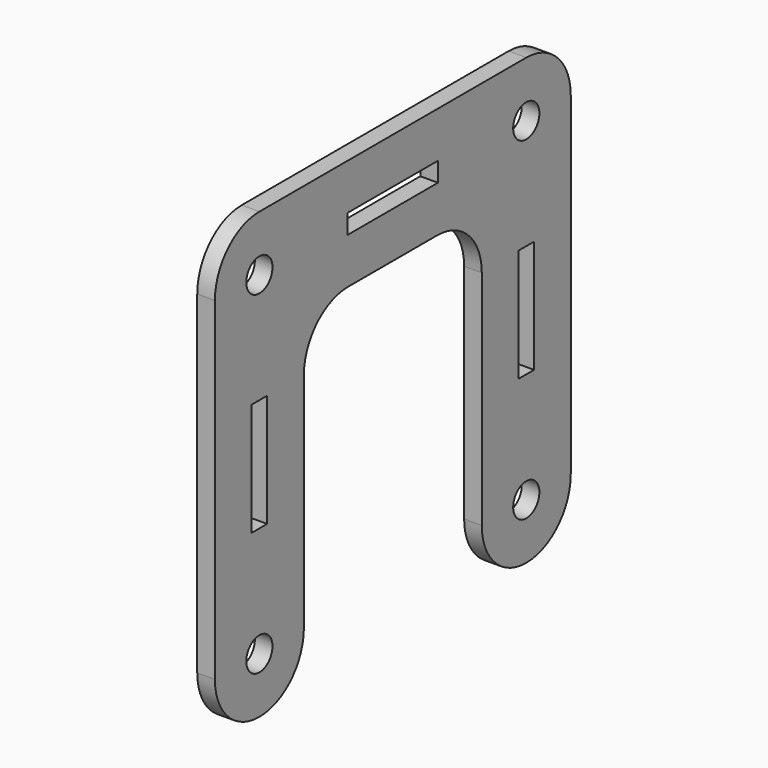
from build123d import *

# Parameters (mm, degrees)
F0_R     = 1.4732
F0_W     = 1.74625
F0_H     = 10.15
F0_W_2   = 10.15
F0_H_2   = 1.74625
F1_DEPTH = 1.5875
F2_R     = 4.99999


# Not quite as in the source:
# - a fillet or chamfer is up to 0.001 mm smaller than in the source, because OpenCascade refuses the exact size
# - a length typed as a fraction of an inch, garbled in the dataset ("3 / 203.2 mm" for 3/8 in), is restored


with BuildPart() as f1:
    # F0 (on Right) → F1 (new body)
    with BuildSketch(Plane.YZ):
        Polygon((20, -20), (20, 20), (-20, 20), (-20, -20), (-10, -20), (-10, 10), (10, 10), (10, -20), align=None)
        with Locations((-15, -15)):
            Circle(F0_R, mode=Mode.SUBTRACT)
        with Locations((15, -15)):
            Circle(F0_R, mode=Mode.SUBTRACT)
        with Locations((-15, 0)):
            Rectangle(F0_W, F0_H, mode=Mode.SUBTRACT)
        with Locations((-15, 15)):
            Circle(F0_R, mode=Mode.SUBTRACT)
        with Locations((15, 0)):
            Rectangle(F0_W, F0_H, mode=Mode.SUBTRACT)
        with Locations((0, 15)):
            Rectangle(F0_W_2, F0_H_2, mode=Mode.SUBTRACT)
        with Locations((15, 15)):
            Circle(F0_R, mode=Mode.SUBTRACT)
    extrude(amount=F1_DEPTH)

    # F2 (radius 5 in the source; OpenCascade refuses exactly that, so slightly less here)
    f2_edges = [f1.edges().sort_by_distance(p)[0] for p in [
        (0.79375, -20, 20),
        (0.79375, -20, -20),
        (0.79375, -10, 10),
        (0.79375, -10, -20),
        (0.79375, 10, -20),
        (0.79375, 20, -20),
        (0.79375, 10, 10),
        (0.79375, 20, 20),
    ]]
    fillet(f2_edges, radius=F2_R)


solid = f1.part
